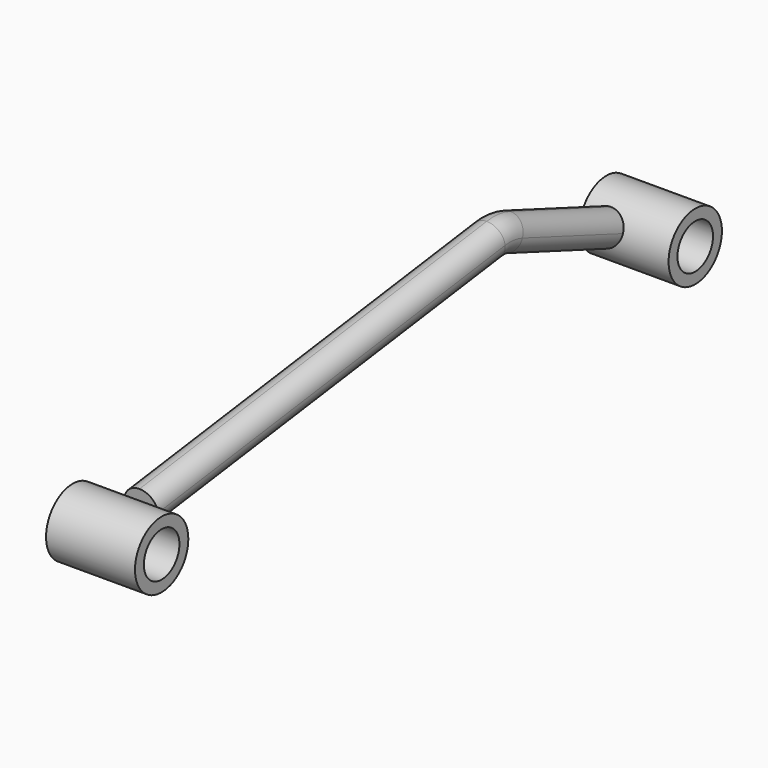
from build123d import *

# Parameters (mm, degrees)
F0_R     = 9.525
F0_R_2   = 6.35
F1_DEPTH = 25.4
F4_DEPTH = 4.7625
F5_R     = 4.76249


# Not quite as in the source:
# - a fillet or chamfer is up to 0.001 mm smaller than in the source, because OpenCascade refuses the exact size


with BuildPart() as f1:
    # F0 (on Right) → F1 (new body)
    with BuildSketch(Plane.YZ):
        Circle(F0_R)
        Circle(F0_R_2, mode=Mode.SUBTRACT)
    extrude(amount=F1_DEPTH)


with BuildPart() as f1b:
    # F0 (on Right) → F1, piece 2 (new body)
    with BuildSketch(Plane.YZ):
        with Locations((190.5, 0)):
            Circle(F0_R)
        with Locations((190.5, 0)):
            Circle(F0_R_2, mode=Mode.SUBTRACT)
    extrude(amount=F1_DEPTH)


with BuildPart() as f4:
    # F3 (on offset) → F4 (new body, symmetric)
    with BuildSketch(Plane.YZ.offset(9.525)):
        with BuildLine():
            Line((11.9400664966, 6.4347663754), (12.5835431405, 1.7159376536))
            Line((12.5835431405, 1.7159376536), (13.2270197717, -3.0028909752))
            Line((13.2270197717, -3.0028909752), (137.1685550482, 13.8982274716))
            ThreePointArc((137.1685550482, 13.8982274716), (139.1251729174, 13.9216162696), (141.0280584284, 13.4656258597))
            Line((141.0280584284, 13.4656258597), (176.9363940543, 0))
            Line((176.9363940543, 0), (178.6086190953, 4.4592667759))
            Line((178.6086190953, 4.4592667759), (180.2808448354, 8.9185354163))
            Line((180.2808448354, 8.9185354163), (144.3725092096, 22.3841612761))
            ThreePointArc((144.3725092096, 22.3841612761), (140.1861610854, 23.3873401779), (135.8816017732, 23.3358848222))
            Line((135.8816017732, 23.3358848222), (11.9400664966, 6.4347663754))
        make_face()
    extrude(amount=F4_DEPTH, both=True)

    # F5 (radius 4.7625 in the source; OpenCascade refuses exactly that, so slightly less here)
    f5_edges = [f4.edges().sort_by_distance(p)[0] for p in [
        (14.2875, 75.197787, 5.447668),
        (14.2875, 73.910834, 14.885326),
        (4.7625, 73.910834, 14.885326),
        (4.7625, 75.197787, 5.447668),
    ]]
    fillet(f5_edges, radius=F5_R)


solid = Compound([f1.part, f1b.part, f4.part])
